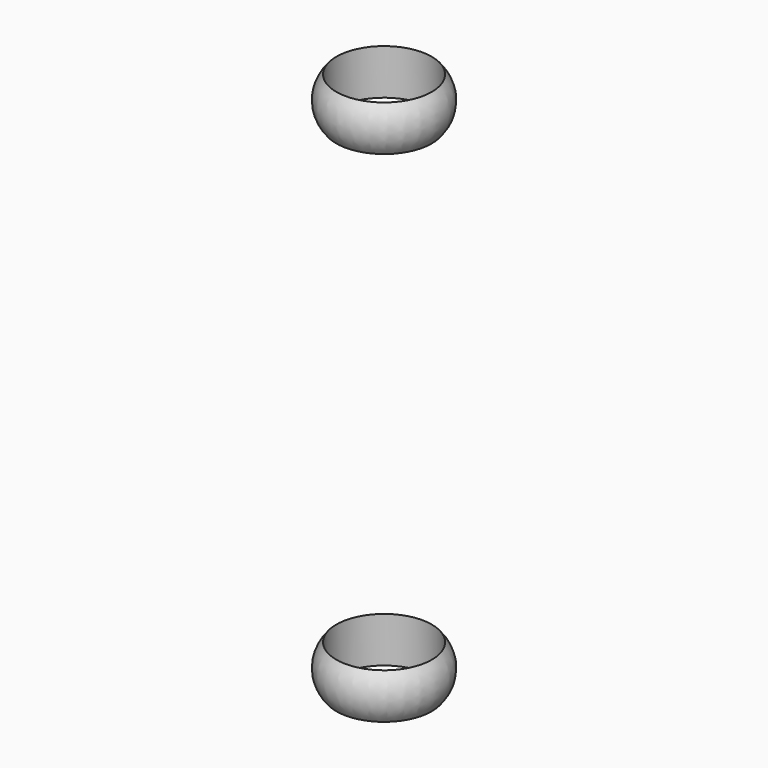
from build123d import *


# Not quite as in the source:
# - the program builds the solid bodies; features that only make, move or delete a surface that nothing else refers to are left out


with BuildPart() as f2:
    # F0 (on Front) → F2 (revolve)
    with BuildSketch(Plane.XZ):
        with BuildLine():
            ThreePointArc((26.67, -57.9410577214), (31.5209683429, -45.2410577214), (26.67, -32.5410577214))
            Line((26.67, -32.5410577214), (26.67, -57.9410577214))
        make_face()
    revolve(axis=Axis((0, 0, 94.4589422786), (0, 0, -1)))


with BuildPart() as f2b:
    # F0 (on Front) → F2, piece 2 (revolve)
    with BuildSketch(Plane.XZ):
        with BuildLine():
            ThreePointArc((26.67, 221.4589422786), (31.5209683429, 234.1589422786), (26.67, 246.8589422786))
            Line((26.67, 246.8589422786), (26.67, 221.4589422786))
        make_face()
    revolve(axis=Axis((0, 0, 94.4589422786), (0, 0, -1)))


solid = Compound([f2.part, f2b.part])
